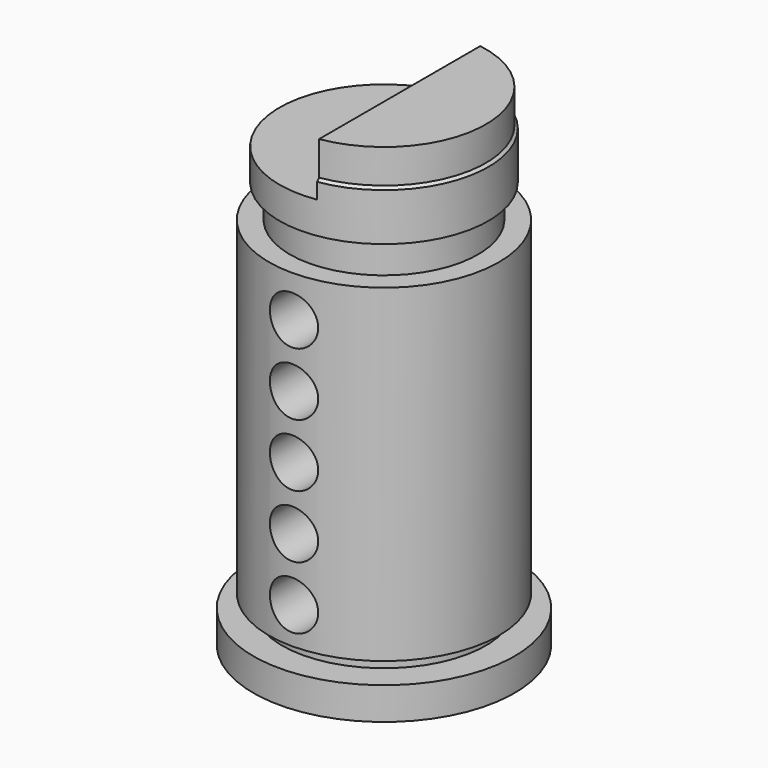
from build123d import *

# Parameters (mm, degrees)
F0_R          = 6.35
F1_DEPTH      = 23.876
F2_R          = 6.35
F2_R_2        = 5.588
F3_DEPTH      = 22.3012
F4_R          = 5.842
F4_R_2        = 4.953
F5_DEPTH      = 0.635
F6_R          = 1.17475
F7_DEPTH      = 5.7404
F7_DEPTH_BACK = 0.0508
F8_R          = 5.715
F8_R_2        = 4.572
F9_DEPTH      = 5.6896
F10_R         = 5.08
F10_R_2       = 4.572
F11_DEPTH     = 4.0894
F12_W         = 7.8048733994
F12_H         = 4.4421355706
F13_DEPTH     = 5.6896
F14_R         = 5.08
F14_R_2       = 4.953
F15_DEPTH     = 1.778
F16_SIZE      = 0.12699
F17_W         = 1.143
F17_H         = 9.652
F18_DEPTH     = 23.877
F19_W         = 1.016
F19_H         = 1.524
F20_DEPTH     = 21.9456
F21_W         = 1.016
F21_H         = 1.5748
F22_DEPTH     = 1.9304
F23_W         = 1.016
F23_H         = 1.778
F24_DEPTH     = 21.336
F25_R         = 0.635
F26_DEPTH     = 21.2852
F29_W         = 1.1630140017
F29_H         = 0.8712620474
F30_DEPTH     = 25.4


# Not quite as in the source:
# - a fillet or chamfer is up to 0.001 mm smaller than in the source, because OpenCascade refuses the exact size


with BuildPart() as f1:
    # F0 (on Top) → F1 (new body)
    with BuildSketch(Plane.XY):
        Circle(F0_R)
    extrude(amount=-F1_DEPTH)

    # F2 (on Top) → F3 (cut)
    with BuildSketch(Plane.XY):
        Circle(F2_R)
        Circle(F2_R_2, mode=Mode.SUBTRACT)
    extrude(amount=-F3_DEPTH, mode=Mode.SUBTRACT)

    # F4 (on face) → F5 (cut)
    with BuildSketch(Plane.XY.offset(-22.3012)):
        Circle(F4_R)
        Circle(F4_R_2, mode=Mode.SUBTRACT)
    extrude(amount=F5_DEPTH, mode=Mode.SUBTRACT)

    # F6 (on Front) → F7 (cut, two sides)
    with BuildSketch(Plane.XZ) as f7_sk:
        with Locations((0, -19.9009)):
            Circle(F6_R)
        with Locations((0, -16.8529)):
            Circle(F6_R)
        with Locations((0, -13.8049)):
            Circle(F6_R)
        with Locations((0, -10.7569)):
            Circle(F6_R)
        with Locations((0, -7.7089)):
            Circle(F6_R)
    extrude(amount=F7_DEPTH, mode=Mode.SUBTRACT)
    extrude(f7_sk.sketch, amount=-F7_DEPTH_BACK, mode=Mode.SUBTRACT)

    # F8 (on face) → F9 (cut, symmetric)
    with BuildSketch(Plane.XY):
        Circle(F8_R)
        Circle(F8_R_2, mode=Mode.SUBTRACT)
    extrude(amount=F9_DEPTH, both=True, mode=Mode.SUBTRACT)

    # F10 (on face) → F11 (join)
    with BuildSketch(Plane.XY):
        Circle(F10_R)
        Circle(F10_R_2, mode=Mode.SUBTRACT)
    extrude(amount=-F11_DEPTH)

    # F12 (on Front) → F13 (cut, symmetric)
    with BuildSketch(Plane.XZ):
        with Locations((-3.1404366997, -0.3189322147)):
            Rectangle(F12_W, F12_H)
    extrude(amount=F13_DEPTH, both=True, mode=Mode.SUBTRACT)

    # F14 (on face) → F15 (cut)
    with BuildSketch(Plane.XY):
        Circle(F14_R)
        Circle(F14_R_2, mode=Mode.SUBTRACT)
    extrude(amount=-F15_DEPTH, mode=Mode.SUBTRACT)

    # F16 (size 0.127 in the source; OpenCascade refuses exactly that, so slightly less here)
    f16_edges = [f1.edges().sort_by_distance(p)[0] for p in [
        (4.953, 0, -1.778),
    ]]
    chamfer(f16_edges, length=F16_SIZE)

    # F17 (on face) → F18 (cut, through all)
    with BuildSketch(Plane(origin=(0, 0, -23.876), x_dir=(1, 0, 0), z_dir=(0, 0, -1))):
        with Locations((0.1905, -1.524)):
            Rectangle(F17_W, F17_H)
    extrude(amount=-F18_DEPTH, mode=Mode.SUBTRACT)

    # F19 (on face) → F20 (cut)
    with BuildSketch(Plane.XY.offset(-2.54)):
        with Locations((-0.889, 4.3036923515)):
            Rectangle(F19_W, F19_H)
    extrude(amount=-F20_DEPTH, mode=Mode.SUBTRACT)

    # F21 (on face) → F22 (cut)
    with BuildSketch(Plane.XZ.offset(-5.0656923515)):
        with Locations((-0.889, -23.0886)):
            Rectangle(F21_W, F21_H)
    extrude(amount=-F22_DEPTH, mode=Mode.SUBTRACT)

    # F23 (on face) → F24 (cut, through all)
    with BuildSketch(Plane.XY.offset(-2.54)):
        with Locations((-0.889, 1.143)):
            Rectangle(F23_W, F23_H)
    extrude(amount=-F24_DEPTH, mode=Mode.SUBTRACT)

    # F25 (on face) → F26 (join)
    with BuildSketch(Plane(origin=(0, 0, -23.876), x_dir=(1, 0, 0), z_dir=(0, 0, -1))):
        with Locations((0.762, -1.27)):
            Circle(F25_R)
    extrude(amount=-F26_DEPTH)

    # F27 (on Right) → F28 (revolve, cut)
    with BuildSketch(Plane.YZ):
        with BuildLine():
            Line((1.4259085423, -23.876), (1.4259085423, -23.368))
            ThreePointArc((1.4259085423, -23.368), (0.2592411198, -23.5154965988), (-0.8600914577, -23.876))
            Line((-0.8600914577, -23.876), (1.4259085423, -23.876))
        make_face()
    revolve(axis=Axis((0, 1.4259085423, -23.622), (0, 0, -1)), mode=Mode.SUBTRACT)

    # F29 (on face) → F30 (cut)
    with BuildSketch(Plane.XY.offset(-5.6896)):
        with Locations((-0.8154929991, 5.274676485)):
            Rectangle(F29_W, F29_H)
    extrude(amount=-F30_DEPTH, mode=Mode.SUBTRACT)


solid = f1.part
